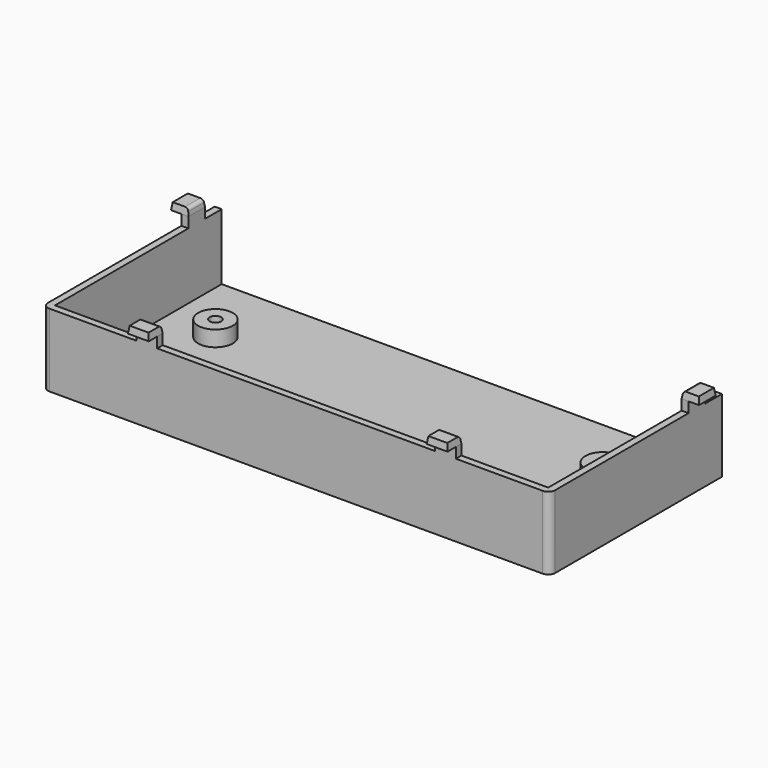
from build123d import *

# Parameters (mm, degrees)
F0_W            = 142
F0_H            = 60
F0_R            = 5
F1_DEPTH        = 19
F2_T            = 2
F3_T1_DEPTH     = 31
F4_W            = 6
F4_H            = 2
F4_W_2          = 2
F4_H_2          = 6
F5_DEPTH        = 3
F6_W            = 5
F6_H            = 6
F6_W_2          = 6
F6_H_2          = 5
F7_DEPTH        = 2
F7_TAPER        = 8
F8_R            = 1
F9_DEPTH        = 4.5
F11_D           = 3.3
F11_CBORE_D     = 6.5
F11_CBORE_DEPTH = 3


# Not quite as in the source:
# - a fillet or chamfer that OpenCascade refuses, or shapes differently, is made with other operations: its cross-section is extruded or revolved along the edge and cut away or added
# - a feature names something its author has since deleted; it is built from what else it names


with BuildPart() as f1:
    # F0 (on Top) → F1 (new body)
    with BuildSketch(Plane.XY):
        Rectangle(F0_W, F0_H)
        with Locations((-50.5, -19)):
            Circle(F0_R, mode=Mode.SUBTRACT)
        with Locations((54.5, -19)):
            Circle(F0_R, mode=Mode.SUBTRACT)
        with Locations((-56, 9)):
            Circle(F0_R, mode=Mode.SUBTRACT)
        with Locations((55.5, 9)):
            Circle(F0_R, mode=Mode.SUBTRACT)
        with Locations((-56, 9)):
            Circle(F0_R)
        with Locations((-50.5, -19)):
            Circle(F0_R)
        with Locations((54.5, -19)):
            Circle(F0_R)
        with Locations((55.5, 9)):
            Circle(F0_R)
    extrude(amount=F1_DEPTH)

    # F2
    f2_openings = [f1.faces().sort_by_distance(p)[0] for p in [
        (0, 0, 19),
        (0, 30, 9.5),
    ]]
    offset(amount=F2_T, openings=f2_openings, kind=Kind.INTERSECTION)

    # F3: fillet of radius 2 on 2 edges, made by hand

    # F3_s2 → F3_t1 (cut)
    with BuildSketch(Plane.XY.offset(-7)):
        with BuildLine():
            ThreePointArc((-71, -32), (-72.4142135624, -31.4142135624), (-73, -30))
            Line((-73, -30), (-73, -32))
            Line((-73, -32), (-71, -32))
        make_face()
        with BuildLine():
            ThreePointArc((71, -32), (72.4142135624, -31.4142135624), (73, -30))
            Line((73, -30), (73, -32))
            Line((73, -32), (71, -32))
        make_face()
    extrude(amount=F3_T1_DEPTH, mode=Mode.SUBTRACT)

    # F4 (on face) → F5 (join)
    with BuildSketch(Plane.XY.offset(19)):
        with Locations((-43, -31)):
            Rectangle(F4_W, F4_H)
        with Locations((-72, 21)):
            Rectangle(F4_W_2, F4_H_2)
        with Locations((72, 21)):
            Rectangle(F4_W_2, F4_H_2)
        with Locations((43, -31)):
            Rectangle(F4_W, F4_H)
    extrude(amount=F5_DEPTH)

    # F6 (on face) → F7 (join)
    with BuildSketch(Plane.XY.offset(22)):
        with Locations((-73.5, 21)):
            Rectangle(F6_W, F6_H)
        with Locations((-43, -32.5)):
            Rectangle(F6_W_2, F6_H_2)
        with Locations((43, -32.5)):
            Rectangle(F6_W_2, F6_H_2)
        with Locations((73.5, 21)):
            Rectangle(F6_W, F6_H)
    extrude(amount=F7_DEPTH, taper=F7_TAPER)

    # F8
    f8_edges = [f1.edges().sort_by_distance(p)[0] for p in [
        (-71.281082, 21, 24),
        (-43, -30.281082, 24),
        (43, -30.281082, 24),
        (71.281082, 21, 24),
    ]]
    fillet(f8_edges, radius=F8_R)

    # F0 (on Top) → F9 (join)
    with BuildSketch(Plane.XY):
        with Locations((-56, 9)):
            Circle(F0_R)
        with Locations((55.5, 9)):
            Circle(F0_R)
        with Locations((54.5, -19)):
            Circle(F0_R)
        with Locations((-50.5, -19)):
            Circle(F0_R)
    extrude(amount=F9_DEPTH)

    # F11 (through all)
    with Locations(Plane(origin=(0, 0, -2), x_dir=(1, 0, 0), z_dir=(0, 0, -1))):
        with Locations((-50.5, 19), (-56, -9), (55.5, -9), (54.5, 19)):
            CounterBoreHole(F11_D / 2, F11_CBORE_D / 2, F11_CBORE_DEPTH)


solid = f1.part
